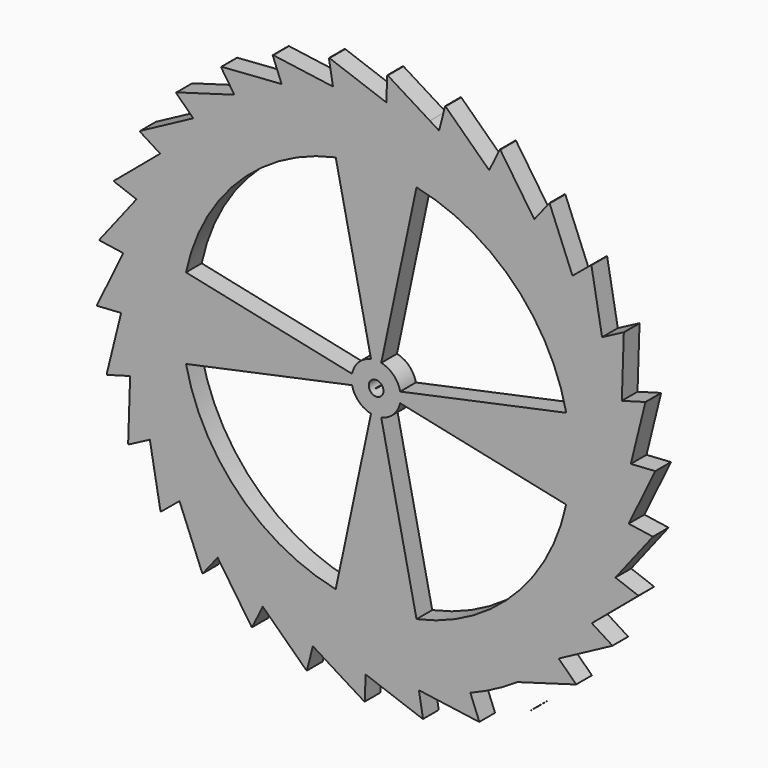
from build123d import *

# Parameters (mm, degrees)
F0_R     = 1.5
F1_DEPTH = 4


with BuildPart() as f1:
    # F0 (on Front) → F1 (new body)
    with BuildSketch(Plane.XZ):
        with BuildLine():
            ThreePointArc((51.423780965, -7.5173518176), (51.8332811532, -3.7685858239), (51.9700209308, 0))
            ThreePointArc((51.9700209308, 0), (51.9431469729, 1.6715769245), (51.8625528764, 3.3414260841))
            ThreePointArc((51.8625528764, 3.3414260841), (51.8624455569, 3.3430923455), (51.8623381838, 3.3447586034))
            ThreePointArc((51.8623381838, 3.3447586034), (51.2287251198, 8.7490139372), (50.0338550026, 14.0574719648))
            ThreePointArc((50.0338550026, 14.0574719648), (50.033403593, 14.0590795014), (50.0329521318, 14.0606870235))
            ThreePointArc((50.0329521318, 14.0606870235), (48.2895771693, 19.2151108485), (46.0171273468, 24.1591388654))
            ThreePointArc((46.0171273468, 24.1591388654), (46.0163515759, 24.1606174201), (46.0155757576, 24.1620959499))
            ThreePointArc((46.0155757576, 24.1620959499), (43.2386327482, 28.8414152114), (39.9879201821, 33.2049354692))
            ThreePointArc((39.9879201821, 33.2049354692), (39.9868539549, 33.2062204221), (39.9857876865, 33.2075053408))
            ThreePointArc((39.9857876865, 33.2075053408), (36.2966423649, 37.2072113331), (32.209738793, 40.799517058))
            ThreePointArc((32.209738793, 40.799517058), (32.2084287087, 40.8005522505), (32.2071185911, 40.801587401))
            ThreePointArc((32.2071185911, 40.801587401), (32.2038705968, 40.8041534125), (32.2006223982, 40.8067191655))
            ThreePointArc((32.2006223982, 40.8067191655), (27.7635059588, 43.9490863386), (23.02252703, 46.6109639736))
            ThreePointArc((23.02252703, 46.6109639736), (23.0210303455, 46.6117041628), (23.0195336373, 46.612444304))
            ThreePointArc((23.0195336373, 46.612444304), (18.0225046976, 48.7658469613), (12.8278101322, 50.3852880993))
            ThreePointArc((12.8278101322, 50.3852880993), (12.8261922599, 50.3857009355), (12.8245743743, 50.3861137196))
            ThreePointArc((12.8245743743, 50.3861137196), (11.8158452876, 50.6327605934), (10.8023920255, 50.8592148629))
            ThreePointArc((10.8023920255, 50.8592148629), (6.4600446281, 51.5934064819), (2.0711461478, 51.9575333597))
            ThreePointArc((2.0711461478, 51.9575333597), (2.0694777965, 51.9576007998), (2.0678094429, 51.9576681863))
            ThreePointArc((2.0678094429, 51.9576681863), (-3.3730714146, 51.892424626), (-8.7773470908, 51.2589850923))
            ThreePointArc((-8.7773470908, 51.2589850923), (-8.7789930063, 51.2587041889), (-8.7806389128, 51.2584232327))
            ThreePointArc((-8.7806389128, 51.2584232327), (-14.0890585705, 50.0633826621), (-19.2435383724, 48.3201732085))
            ThreePointArc((-19.2435383724, 48.3201732085), (-19.2450899176, 48.3195562385), (-19.246641443, 48.3189392186))
            ThreePointArc((-19.246641443, 48.3189392186), (-24.1905964893, 46.0463306451), (-28.8700049156, 43.2695378896))
            ThreePointArc((-28.8700049156, 43.2695378896), (-28.8713942805, 43.2686118174), (-28.8727836157, 43.2676857006))
            ThreePointArc((-28.8727836157, 43.2676857006), (-33.2361994913, 40.0168330241), (-37.2360239395, 36.3278161346))
            ThreePointArc((-37.2360239395, 36.3278161346), (-37.2371904022, 36.3266214341), (-37.2383568266, 36.3254266962))
            ThreePointArc((-37.2383568266, 36.3254266962), (-40.8305313197, 32.2384077779), (-43.9759602681, 27.7983944943))
            ThreePointArc((-43.9759602681, 27.7983944943), (-43.9768528486, 27.7969833797), (-43.9777453839, 27.7955722364))
            ThreePointArc((-43.9777453839, 27.7955722364), (-46.641683232, 23.0510094147), (-48.7952463421, 18.0540496231))
            ThreePointArc((-48.7952463421, 18.0540496231), (-48.7958260304, 18.0524837668), (-48.7964056684, 18.0509178919))
            ThreePointArc((-48.7964056684, 18.0509178919), (-50.4156800046, 12.8561713291), (-51.4832562346, 7.5206561505))
            ThreePointArc((-51.4832562346, 7.5206561505), (-51.4834976955, 7.5190039879), (-51.4837391033, 7.5173518176))
            ThreePointArc((-51.4837391033, 7.5173518176), (-51.9875798689, 2.0994568656), (-51.9225110148, -3.341426084))
            ThreePointArc((-51.9225110148, -3.341426084), (-51.9224036952, -3.3430923454), (-51.9222963221, -3.3447586034))
            ThreePointArc((-51.9222963221, -3.3447586034), (-51.2886832581, -8.7490139372), (-50.0938131409, -14.0574719648))
            ThreePointArc((-50.0938131409, -14.0574719648), (-50.0933617313, -14.0590795013), (-50.0929102701, -14.0606870234))
            ThreePointArc((-50.0929102701, -14.0606870234), (-48.3495353076, -19.2151108485), (-46.0770854851, -24.1591388654))
            ThreePointArc((-46.0770854851, -24.1591388654), (-46.0763097143, -24.1606174201), (-46.0755338959, -24.1620959499))
            ThreePointArc((-46.0755338959, -24.1620959499), (-43.2985908866, -28.8414152114), (-40.0478783205, -33.2049354692))
            ThreePointArc((-40.0478783205, -33.2049354692), (-40.0468120933, -33.2062204221), (-40.0457458248, -33.2075053408))
            ThreePointArc((-40.0457458248, -33.2075053408), (-36.3566005033, -37.207211333), (-32.2696969313, -40.799517058))
            ThreePointArc((-32.2696969313, -40.799517058), (-32.268386847, -40.8005522505), (-32.2670767295, -40.801587401))
            ThreePointArc((-32.2670767295, -40.801587401), (-27.8269624488, -43.9468737795), (-23.0824851683, -46.6109639736))
            ThreePointArc((-23.0824851683, -46.6109639736), (-23.0809884839, -46.6117041628), (-23.0794917756, -46.612444304))
            ThreePointArc((-23.0794917756, -46.612444304), (-18.082462836, -48.7658469613), (-12.8877682706, -50.3852880993))
            ThreePointArc((-12.8877682706, -50.3852880993), (-12.8861503982, -50.3857009355), (-12.8845325127, -50.3861137196))
            ThreePointArc((-12.8845325127, -50.3861137196), (-7.5489830571, -51.4535186263), (-2.1311042862, -51.9575333597))
            ThreePointArc((-2.1311042862, -51.9575333597), (-2.1294359348, -51.9576007998), (-2.1277675813, -51.9576681863))
            ThreePointArc((-2.1277675813, -51.9576681863), (3.3131132763, -51.892424626), (8.7173889525, -51.2589850923))
            ThreePointArc((8.7173889525, -51.2589850923), (8.719034868, -51.2587041889), (8.7206807744, -51.2584232327))
            ThreePointArc((8.7206807744, -51.2584232327), (14.0291004322, -50.0633826621), (19.1835802341, -48.3201732085))
            ThreePointArc((19.1835802341, -48.3201732085), (19.1851317793, -48.3195562385), (19.1866833047, -48.3189392186))
            ThreePointArc((19.1866833047, -48.3189392186), (24.1306383509, -46.0463306451), (28.8100467773, -43.2695378896))
            ThreePointArc((28.8100467773, -43.2695378896), (28.8114361422, -43.2686118174), (28.8128254774, -43.2676857007))
            ThreePointArc((28.8128254774, -43.2676857007), (33.1762413529, -40.0168330241), (37.1760658011, -36.3278161346))
            ThreePointArc((37.1760658011, -36.3278161346), (37.1772322639, -36.3266214341), (37.1783986882, -36.3254266962))
            ThreePointArc((37.1783986882, -36.3254266962), (40.7705731814, -32.2384077779), (43.9160021298, -27.7983944943))
            ThreePointArc((43.9160021298, -27.7983944943), (43.9168947103, -27.7969833797), (43.9177872455, -27.7955722364))
            ThreePointArc((43.9177872455, -27.7955722364), (46.5817250937, -23.0510094147), (48.7352882038, -18.0540496231))
            ThreePointArc((48.7352882038, -18.0540496231), (48.7358678921, -18.0524837668), (48.7364475301, -18.0509178919))
            ThreePointArc((48.7364475301, -18.0509178919), (50.3557218663, -12.8561713291), (51.4232980963, -7.5206561505))
            ThreePointArc((51.4232980963, -7.5206561505), (51.4235395572, -7.5190039879), (51.423780965, -7.5173518176))
        make_face()
        with BuildLine():
            Line((-38.7123002544, -8.1905973513), (-4.8907380037, -1.001602369))
            ThreePointArc((-4.8907380037, -1.001602369), (-3.535533906, -3.4975778209), (-1.0395584541, -4.8527819186))
            Line((-1.0395584541, -4.8527819186), (-8.2285534364, -38.6743441693))
            ThreePointArc((-8.2285534364, -38.6743441693), (-27.9852754377, -27.9473193526), (-38.7123002544, -8.1905973513))
        make_face(mode=Mode.SUBTRACT)
        with BuildLine():
            ThreePointArc((1.0395584541, -4.8527819186), (3.5201705738, -3.5128746813), (4.881539124, -1.0439754197))
            Line((4.881539124, -1.0439754197), (38.7032620429, -8.2330045531))
            ThreePointArc((38.7032620429, -8.2330045531), (27.9699412844, -27.9626451083), (8.2285534364, -38.6743441693))
            Line((8.2285534364, -38.6743441693), (1.0395584541, -4.8527819186))
        make_face(mode=Mode.SUBTRACT)
        with Locations((0, 0.037956085)):
            Circle(F0_R, mode=Mode.SUBTRACT)
        with BuildLine():
            ThreePointArc((-38.7212920003, 8.2240924432), (-28.0006011933, 28.0078973695), (-8.2285534364, 38.7502563394))
            Line((-8.2285534364, 38.7502563394), (-1.0395584541, 4.9286940887))
            ThreePointArc((-1.0395584541, 4.9286940887), (-3.5508307664, 3.5581266589), (-4.8995690813, 1.0350633097))
            Line((-4.8995690813, 1.0350633097), (-38.7212920003, 8.2240924432))
        make_face(mode=Mode.SUBTRACT)
        with BuildLine():
            ThreePointArc((4.8983222404, 1.0411705334), (3.5486358835, 3.5603392792), (1.0395584541, 4.9286940887))
            Line((1.0395584541, 4.9286940887), (8.2285534364, 38.7502563394))
            ThreePointArc((8.2285534364, 38.7502563394), (27.9983986149, 28.0101021886), (38.7200022863, 8.2301905538))
            Line((38.7200022863, 8.2301905538), (4.8983222404, 1.0411705334))
        make_face(mode=Mode.SUBTRACT)
        with BuildLine():
            ThreePointArc((51.8625528764, 3.3414260841), (51.9431469729, 1.6715769245), (51.9700209308, 0))
            ThreePointArc((51.9700209308, 0), (51.8332811532, -3.7685858239), (51.423780965, -7.5173518176))
            Line((51.423780965, -7.5173518176), (51.4248273891, -7.5175046993))
            Line((51.4248273891, -7.5175046993), (56.8415524882, 3.6448733841))
            ThreePointArc((56.8415524882, 3.6448733841), (56.8408849757, 3.6552424829), (56.8402155713, 3.6656114598))
            Line((56.8402155713, 3.6656114598), (51.863393527, 3.3448266263))
            Line((51.863393527, 3.3448266263), (51.8625528764, 3.3414260841))
        make_face()
        with BuildLine():
            ThreePointArc((51.8623381838, 3.3447586034), (51.8624455569, 3.3430923455), (51.8625528764, 3.3414260841))
            Line((51.8625528764, 3.3414260841), (51.863393527, 3.3448266263))
            Line((51.863393527, 3.3448266263), (51.8623381838, 3.3447586034))
        make_face()
        with BuildLine():
            Line((51.4248273891, -7.5175046993), (51.423780965, -7.5173518176))
            ThreePointArc((51.423780965, -7.5173518176), (51.4235395572, -7.5190039879), (51.4232980963, -7.5206561505))
            Line((51.4232980963, -7.5206561505), (51.4248273891, -7.5175046993))
        make_face()
        with BuildLine():
            ThreePointArc((50.0338550026, 14.0574719648), (51.2287251198, 8.7490139372), (51.8623381838, 3.3447586034))
            Line((51.8623381838, 3.3447586034), (51.863393527, 3.3448266263))
            Line((51.863393527, 3.3448266263), (54.8394310956, 15.383290621))
            ThreePointArc((54.8394310956, 15.383290621), (54.8358719487, 15.3959636245), (54.8323098726, 15.4086358049))
            Line((54.8323098726, 15.4086358049), (50.0339702704, 14.0609729781))
            Line((50.0339702704, 14.0609729781), (50.0338550025, 14.0574719648))
        make_face()
        with BuildLine():
            Line((51.4248273891, -7.5175046993), (51.4232980963, -7.5206561505))
            ThreePointArc((51.4232980963, -7.5206561505), (50.3557218663, -12.8561713291), (48.7364475301, -18.0509178919))
            Line((48.7364475301, -18.0509178919), (48.7374393014, -18.0512849966))
            Line((48.7374393014, -18.0512849966), (56.3583664405, -8.2567424152))
            ThreePointArc((56.3583664405, -8.2567424152), (56.3596879193, -8.2477096133), (56.3610079501, -8.2386765998))
            Line((56.3610079501, -8.2386765998), (51.4248273891, -7.5175046993))
        make_face()
        with BuildLine():
            ThreePointArc((50.0329521318, 14.0606870235), (50.033403593, 14.0590795014), (50.0338550026, 14.0574719648))
            Line((50.0338550025, 14.0574719648), (50.0339702704, 14.0609729781))
            Line((50.0339702704, 14.0609729781), (50.0329521318, 14.0606870235))
        make_face()
        with BuildLine():
            Line((48.7374393014, -18.0512849966), (48.7364475301, -18.0509178919))
            ThreePointArc((48.7364475301, -18.0509178919), (48.7358678921, -18.0524837668), (48.7352882038, -18.0540496231))
            Line((48.7352882038, -18.0540496231), (48.7374393014, -18.0512849966))
        make_face()
        with BuildLine():
            ThreePointArc((46.0171273468, 24.1591388654), (48.2895771693, 19.2151108485), (50.0329521318, 14.0606870235))
            Line((50.0329521318, 14.0606870235), (50.0339702704, 14.0609729781))
            Line((50.0339702704, 14.0609729781), (50.4417219085, 26.4455542565))
            ThreePointArc((50.4417219085, 26.4455542565), (50.4336714583, 26.4608959315), (50.425616341, 26.4762351567))
            Line((50.425616341, 26.4762351567), (46.0165121942, 24.1625873387))
            Line((46.0165121942, 24.1625873387), (46.0171273468, 24.1591388654))
        make_face()
        with BuildLine():
            Line((48.7374393014, -18.0512849966), (48.7352882038, -18.0540496231))
            ThreePointArc((48.7352882038, -18.0540496231), (46.5817250937, -23.0510094147), (43.9177872455, -27.7955722364))
            Line((43.9177872455, -27.7955722364), (43.918681019, -27.7961375198))
            Line((43.918681019, -27.7961375198), (53.4089351369, -19.8005617916))
            ThreePointArc((53.4089351369, -19.8005617916), (53.4122132861, -19.7917150962), (53.4154899695, -19.7828678578))
            Line((53.4154899695, -19.7828678579), (48.7374393014, -18.0512849966))
        make_face()
        with BuildLine():
            ThreePointArc((46.0155757576, 24.1620959499), (46.0163515759, 24.1606174201), (46.0171273468, 24.1591388654))
            Line((46.0171273468, 24.1591388654), (46.0165121942, 24.1625873387))
            Line((46.0165121942, 24.1625873387), (46.0155757576, 24.1620959499))
        make_face()
        with BuildLine():
            Line((43.918681019, -27.7961375198), (43.9177872455, -27.7955722364))
            ThreePointArc((43.9177872455, -27.7955722364), (43.9168947103, -27.7969833797), (43.9160021298, -27.7983944943))
            Line((43.9160021298, -27.7983944943), (43.918681019, -27.7961375198))
        make_face()
        with BuildLine():
            ThreePointArc((39.9879201821, 33.2049354692), (43.2386327482, 28.8414152114), (46.0155757576, 24.1620959499))
            Line((46.0155757576, 24.1620959499), (46.0165121942, 24.1625873387))
            Line((46.0165121942, 24.1625873387), (43.8426229041, 36.349154898))
            ThreePointArc((43.8426229041, 36.349154898), (43.8281298887, 36.3666205946), (43.8136299139, 36.384080514))
            Line((43.8136299139, 36.384080514), (39.9866014941, 33.2081806877))
            Line((39.9866014941, 33.2081806877), (39.9879201821, 33.2049354692))
        make_face()
        with BuildLine():
            Line((43.918681019, -27.7961375198), (43.9160021298, -27.7983944943))
            ThreePointArc((43.9160021298, -27.7983944943), (40.7705731814, -32.2384077779), (37.1783986882, -36.3254266962))
            Line((37.1783986883, -36.3254266962), (37.1791554016, -36.3261654528))
            Line((37.1791554016, -36.3261654528), (48.1206244533, -30.4804633073))
            ThreePointArc((48.1206244533, -30.4804633073), (48.1266672862, -30.4709204774), (48.1327082262, -30.4613764493))
            Line((48.1327082262, -30.4613764493), (43.918681019, -27.7961375198))
        make_face()
        with BuildLine():
            ThreePointArc((39.9857876865, 33.2075053408), (39.9868539549, 33.2062204221), (39.9879201821, 33.2049354692))
            Line((39.9879201821, 33.2049354692), (39.9866014941, 33.2081806877))
            Line((39.9866014941, 33.2081806877), (39.9857876865, 33.2075053408))
        make_face()
        with BuildLine():
            Line((37.1791554016, -36.3261654528), (37.1783986883, -36.3254266962))
            ThreePointArc((37.1783986882, -36.3254266962), (37.1772322639, -36.3266214341), (37.1760658011, -36.3278161346))
            Line((37.1760658011, -36.3278161346), (37.1791554016, -36.3261654528))
        make_face()
        with BuildLine():
            ThreePointArc((32.209738793, 40.799517058), (36.2966423649, 37.2072113331), (39.9857876865, 33.2075053408))
            Line((39.9857876865, 33.2075053408), (39.9866014941, 33.2081806877))
            Line((39.9866014941, 33.2081806877), (35.3319790375, 44.662949992))
            ThreePointArc((35.3319790375, 44.662949992), (35.3091952691, 44.6809558924), (35.286402322, 44.6989501724))
            Line((35.286402322, 44.6989501724), (32.2091226063, 40.8041238266))
            Line((32.2091226063, 40.8041238266), (32.209738793, 40.799517058))
        make_face()
        with BuildLine():
            Line((37.1791554016, -36.3261654528), (37.1760658011, -36.3278161346))
            ThreePointArc((37.1760658011, -36.3278161346), (33.1762413529, -40.0168330241), (28.8128254774, -43.2676857007))
            Line((28.8128254774, -43.2676857007), (28.8134120585, -43.2685656432))
            Line((28.8134120585, -43.2685656432), (40.7238038627, -39.8275945924))
            ThreePointArc((40.7238038627, -39.8275945924), (40.7340326593, -39.8171332475), (40.7442587679, -39.8066692749))
            Line((40.7442587679, -39.8066692749), (37.1791554016, -36.3261654528))
        make_face()
        with BuildLine():
            ThreePointArc((32.2071185911, 40.801587401), (32.2084287087, 40.8005522505), (32.209738793, 40.799517058))
            Line((32.209738793, 40.799517058), (32.2077742026, 40.80241719))
            Line((32.2077742026, 40.80241719), (32.2071185911, 40.801587401))
        make_face()
        Polygon((32.2077742026, 40.80241719), (32.209738793, 40.799517058), (32.2091226063, 40.8041238266), align=None)
        with BuildLine():
            Line((28.8134120585, -43.2685656432), (28.8128254774, -43.2676857007))
            ThreePointArc((28.8128254774, -43.2676857007), (28.8114361422, -43.2686118174), (28.8100467773, -43.2695378896))
            Line((28.8100467773, -43.2695378896), (28.8134120585, -43.2685656432))
        make_face()
        with BuildLine():
            ThreePointArc((32.2006223982, 40.8067191655), (32.2038705968, 40.8041534125), (32.2071185911, 40.801587401))
            Line((32.2071185911, 40.801587401), (32.2077742026, 40.80241719))
            Line((32.2077742026, 40.80241719), (32.2029035341, 40.8096072802))
            Line((32.2029035341, 40.8096072802), (32.2006223982, 40.8067191655))
        make_face()
        Polygon((32.2029035341, 40.8096072802), (32.2077742026, 40.80241719), (32.2091226063, 40.8041238266), (32.2075947163, 40.8155467211), align=None)
        with BuildLine():
            ThreePointArc((23.02252703, 46.6109639736), (27.7635059588, 43.9490863386), (32.2006223982, 40.8067191655))
            Line((32.2006223982, 40.8067191655), (32.2029035341, 40.8096072802))
            Line((32.2029035341, 40.8096072802), (25.282367975, 51.0257149897))
            ThreePointArc((25.282367975, 51.0257149897), (25.2500286651, 51.0417168963), (25.2176792232, 51.0576983102))
            Line((25.2176792232, 51.0576983102), (23.0200023993, 46.6133922695))
            Line((23.0200023993, 46.6133922695), (23.02252703, 46.6109639736))
        make_face()
        with BuildLine():
            Line((19.1870741173, -48.3199218894), (19.1866833047, -48.3189392186))
            ThreePointArc((19.1866833047, -48.3189392186), (19.1851317793, -48.3195562385), (19.1835802341, -48.3201732085))
            Line((19.1835802341, -48.3201732085), (19.1870741173, -48.3199218894))
        make_face()
        with BuildLine():
            ThreePointArc((23.0195336373, 46.612444304), (23.0210303455, 46.6117041628), (23.02252703, 46.6109639736))
            Line((23.02252703, 46.6109639736), (23.0200023993, 46.6133922695))
            Line((23.0200023993, 46.6133922695), (23.0195336373, 46.612444304))
        make_face()
        with BuildLine():
            Line((19.1870741173, -48.3199218894), (19.1835802341, -48.3201732085))
            ThreePointArc((19.1835802341, -48.3201732085), (14.0291004322, -50.0633826621), (8.7206807744, -51.2584232327))
            Line((8.7206807744, -51.2584232327), (8.7208587382, -51.2594656842))
            Line((8.7208587382, -51.2594656842), (20.9772836713, -52.9570745732))
            ThreePointArc((20.9772836713, -52.9570745732), (21.0006110859, -52.9478310737), (21.0239344255, -52.9385772969))
            Line((21.0239344255, -52.9385772969), (19.1870741173, -48.3199218894))
        make_face()
        with BuildLine():
            ThreePointArc((12.8278101322, 50.3852880993), (18.0225046976, 48.7658469613), (23.0195336373, 46.612444304))
            Line((23.0195336373, 46.612444304), (23.0200023993, 46.6133922695))
            Line((23.0200023993, 46.6133922695), (14.1327095736, 55.1615638726))
            ThreePointArc((14.1327095736, 55.1615638726), (14.0905496682, 55.1723391221), (14.0483815417, 55.1830821538))
            Line((14.0483815417, 55.1830821538), (12.8248357996, 50.3871384309))
            Line((12.8248357996, 50.3871384309), (12.8278101322, 50.3852880993))
        make_face()
        with BuildLine():
            Line((8.7208587382, -51.2594656842), (8.7206807744, -51.2584232327))
            ThreePointArc((8.7206807744, -51.2584232327), (8.719034868, -51.2587041889), (8.7173889525, -51.2589850923))
            Line((8.7173889525, -51.2589850923), (8.7208587382, -51.2594656842))
        make_face()
        with BuildLine():
            ThreePointArc((12.8245743743, 50.3861137196), (12.8261922599, 50.3857009355), (12.8278101322, 50.3852880993))
            Line((12.8278101322, 50.3852880993), (12.8248357996, 50.3871384309))
            Line((12.8248357996, 50.3871384309), (12.8245743743, 50.3861137196))
        make_face()
        with BuildLine():
            Line((8.7208587382, -51.2594656842), (8.7173889525, -51.2589850923))
            ThreePointArc((8.7173889525, -51.2589850923), (3.3131132763, -51.892424626), (-2.1277675813, -51.9576681863))
            Line((-2.1277675813, -51.9576681863), (-2.1278102444, -51.9587248585))
            Line((-2.1278102444, -51.9587248585), (9.4934072875, -56.1622741859))
            ThreePointArc((9.4934072875, -56.1622741859), (9.5247237806, -56.1569763154), (9.5560373141, -56.1516609799))
            Line((9.5560373141, -56.1516609799), (8.7208587382, -51.2594656842))
        make_face()
        with BuildLine():
            ThreePointArc((10.8023920255, 50.8592148629), (11.8158452876, 50.6327605934), (12.8245743743, 50.3861137196))
            Line((12.8245743743, 50.3861137196), (12.8248357996, 50.3871384309))
            Line((12.8248357996, 50.3871384309), (10.949965744, 51.5534946223))
            Line((10.949965744, 51.5534946223), (10.8023920255, 50.8592148629))
        make_face()
        with BuildLine():
            Line((-2.1278102444, -51.9587248585), (-2.1277675813, -51.9576681863))
            ThreePointArc((-2.1277675813, -51.9576681863), (-2.1294359348, -51.9576007998), (-2.1311042862, -51.9575333597))
            Line((-2.1311042862, -51.9575333597), (-2.1278102444, -51.9587248585))
        make_face()
        with BuildLine():
            ThreePointArc((2.0711461478, 51.9575333597), (6.4600446281, 51.5934064819), (10.8023920255, 50.8592148629))
            Line((10.8023920255, 50.8592148629), (10.949965744, 51.5534946223))
            Line((10.949965744, 51.5534946223), (2.3691338098, 56.8916280168))
            ThreePointArc((2.3691338098, 56.8916280168), (2.318160244, 56.8937186784), (2.2671848258, 56.8957636756))
            Line((2.2671848258, 56.8957636756), (2.067852106, 51.9587248585))
            Line((2.067852106, 51.9587248585), (2.0711461478, 51.9575333597))
        make_face()
        with BuildLine():
            Line((-2.1278102444, -51.9587248585), (-2.1311042862, -51.9575333597))
            ThreePointArc((-2.1311042862, -51.9575333597), (-7.5489830571, -51.4535186263), (-12.8845325127, -50.3861137196))
            Line((-12.8845325127, -50.3861137196), (-12.884793938, -50.3871384309))
            Line((-12.884793938, -50.3871384309), (-2.4056567842, -56.9062070265))
            ThreePointArc((-2.4056567842, -56.9062070265), (-2.3666769917, -56.9078484907), (-2.3276960839, -56.9094632505))
            Line((-2.3276960839, -56.9094632505), (-2.1278102444, -51.9587248585))
        make_face()
        with BuildLine():
            ThreePointArc((2.0678094429, 51.9576681863), (2.0694777965, 51.9576007998), (2.0711461478, 51.9575333597))
            Line((2.0711461478, 51.9575333597), (2.067852106, 51.9587248585))
            Line((2.067852106, 51.9587248585), (2.0678094429, 51.9576681863))
        make_face()
        with BuildLine():
            Line((-12.884793938, -50.3871384309), (-12.8845325127, -50.3861137196))
            ThreePointArc((-12.8845325127, -50.3861137196), (-12.8861503982, -50.3857009355), (-12.8877682706, -50.3852880993))
            Line((-12.8877682706, -50.3852880993), (-12.884793938, -50.3871384309))
        make_face()
        with BuildLine():
            ThreePointArc((-8.7773470908, 51.2589850923), (-3.3730714146, 51.892424626), (2.0678094429, 51.9576681863))
            Line((2.0678094429, 51.9576681863), (2.067852106, 51.9587248585))
            Line((2.067852106, 51.9587248585), (-9.4960653121, 56.1415479707))
            ThreePointArc((-9.4960653121, 56.1415479707), (-9.553501977, 56.1317939904), (-9.6109286334, 56.1219812573))
            Line((-9.6109286334, 56.1219812573), (-8.7808168765, 51.2594656842))
            Line((-8.7808168765, 51.2594656842), (-8.7773470908, 51.2589850923))
        make_face()
        with BuildLine():
            Line((-12.884793938, -50.3871384309), (-12.8877682706, -50.3852880993))
            ThreePointArc((-12.8877682706, -50.3852880993), (-18.082462836, -48.7658469613), (-23.0794917756, -46.612444304))
            Line((-23.0794917756, -46.612444304), (-23.0799605376, -46.6133922695))
            Line((-23.0799605376, -46.6133922695), (-14.1976694582, -55.1567529829))
            ThreePointArc((-14.1976694582, -55.1567529829), (-14.1526030357, -55.1683435564), (-14.1075271576, -55.1798973022))
            Line((-14.1075271576, -55.1798973022), (-12.884793938, -50.3871384309))
        make_face()
        with BuildLine():
            ThreePointArc((-8.7806389128, 51.2584232327), (-8.7789930063, 51.2587041889), (-8.7773470908, 51.2589850923))
            Line((-8.7773470908, 51.2589850923), (-8.7808168765, 51.2594656842))
            Line((-8.7808168765, 51.2594656842), (-8.7806389128, 51.2584232327))
        make_face()
        with BuildLine():
            Line((-23.0799605376, -46.6133922695), (-23.0794917756, -46.612444304))
            ThreePointArc((-23.0794917756, -46.612444304), (-23.0809884839, -46.6117041628), (-23.0824851683, -46.6109639736))
            Line((-23.0824851683, -46.6109639736), (-23.0799605376, -46.6133922695))
        make_face()
        with BuildLine():
            ThreePointArc((-19.2435383724, 48.3201732085), (-14.0890585705, 50.0633826621), (-8.7806389128, 51.2584232327))
            Line((-8.7806389128, 51.2584232327), (-8.7808168765, 51.2594656842))
            Line((-8.7808168765, 51.2594656842), (-20.9465042524, 52.9445067253))
            ThreePointArc((-20.9465042524, 52.9445067253), (-21.0068617668, 52.9205801703), (-21.0671919636, 52.8965848179))
            Line((-21.0671919636, 52.8965848179), (-19.2470322556, 48.3199218893))
            Line((-19.2470322556, 48.3199218893), (-19.2435383724, 48.3201732085))
        make_face()
        with BuildLine():
            Line((-23.0799605376, -46.6133922695), (-23.0824851683, -46.6109639736))
            ThreePointArc((-23.0824851683, -46.6109639736), (-27.8269624488, -43.9468737795), (-32.2670767295, -40.801587401))
            Line((-32.2670767295, -40.801587401), (-32.267732341, -40.80241719))
            Line((-32.267732341, -40.80241719), (-25.3654197169, -50.9916241683))
            ThreePointArc((-25.3654197169, -50.9916241683), (-25.3170761133, -51.0156571166), (-25.2687097482, -51.0396442242))
            Line((-25.2687097482, -51.0396442242), (-23.0799605376, -46.6133922695))
        make_face()
        with BuildLine():
            ThreePointArc((-19.246641443, 48.3189392186), (-19.2450899176, 48.3195562385), (-19.2435383724, 48.3201732085))
            Line((-19.2435383724, 48.3201732085), (-19.2470322556, 48.3199218893))
            Line((-19.2470322556, 48.3199218893), (-19.246641443, 48.3189392186))
        make_face()
        with BuildLine():
            Line((-32.267732341, -40.80241719), (-32.2670767295, -40.801587401))
            ThreePointArc((-32.2670767295, -40.801587401), (-32.268386847, -40.8005522505), (-32.2696969313, -40.799517058))
            Line((-32.2696969314, -40.799517058), (-32.267732341, -40.80241719))
        make_face()
        with BuildLine():
            ThreePointArc((-28.8700049156, 43.2695378896), (-24.1905964893, 46.0463306451), (-19.246641443, 48.3189392186))
            Line((-19.246641443, 48.3189392186), (-19.2470322556, 48.3199218893))
            Line((-19.2470322556, 48.3199218893), (-31.4839020622, 47.4397093574))
            ThreePointArc((-31.4839020622, 47.4397093574), (-31.5428070152, 47.4005584273), (-31.6016632984, 47.3613343691))
            Line((-31.6016632984, 47.3613343691), (-28.8733701969, 43.2685656432))
            Line((-28.8733701969, 43.2685656432), (-28.8700049156, 43.2695378896))
        make_face()
        with BuildLine():
            Line((-32.267732341, -40.80241719), (-32.2696969314, -40.799517058))
            ThreePointArc((-32.2696969313, -40.799517058), (-36.3566005033, -37.207211333), (-40.0457458248, -33.2075053408))
            Line((-40.0457458248, -33.2075053408), (-40.0465596325, -33.2081806877))
            Line((-40.0465596325, -33.2081806877), (-35.4196493073, -44.5947519638))
            ThreePointArc((-35.4196493073, -44.5947519638), (-35.3718307251, -44.6327081594), (-35.3239714799, -44.6706130698))
            Line((-35.3239714799, -44.6706130698), (-32.267732341, -40.80241719))
        make_face()
        with BuildLine():
            ThreePointArc((-28.8727836157, 43.2676857006), (-28.8713942805, 43.2686118174), (-28.8700049156, 43.2695378896))
            Line((-28.8700049156, 43.2695378896), (-28.8733701969, 43.2685656432))
            Line((-28.8733701969, 43.2685656432), (-28.8727836157, 43.2676857006))
        make_face()
        with BuildLine():
            Line((-40.0465596325, -33.2081806877), (-40.0457458248, -33.2075053408))
            ThreePointArc((-40.0457458248, -33.2075053408), (-40.0468120933, -33.2062204221), (-40.0478783205, -33.2049354692))
            Line((-40.0478783205, -33.2049354692), (-40.0465596325, -33.2081806877))
        make_face()
        with BuildLine():
            ThreePointArc((-37.2360239395, 36.3278161346), (-33.2361994913, 40.0168330241), (-28.8727836157, 43.2676857006))
            Line((-28.8727836157, 43.2676857006), (-28.8733701969, 43.2685656432))
            Line((-28.8733701969, 43.2685656432), (-40.6494848981, 39.866387911))
            ThreePointArc((-40.6494848981, 39.866387911), (-40.702250937, 39.8125124482), (-40.7549455886, 39.7585671606))
            Line((-40.7549455886, 39.7585671606), (-37.2391135399, 36.3261654528))
            Line((-37.2391135399, 36.3261654528), (-37.2360239395, 36.3278161346))
        make_face()
        with BuildLine():
            Line((-40.0465596325, -33.2081806877), (-40.0478783205, -33.2049354692))
            ThreePointArc((-40.0478783205, -33.2049354692), (-43.2985908866, -28.8414152114), (-46.0755338959, -24.1620959499))
            Line((-46.0755338959, -24.1620959499), (-46.0764703325, -24.1625873387))
            Line((-46.0764703325, -24.1625873387), (-43.9206397604, -36.2479198503))
            ThreePointArc((-43.9206397604, -36.2479198503), (-43.8777101404, -36.2998976723), (-43.8347190213, -36.3518246394))
            Line((-43.8347190213, -36.3518246394), (-40.0465596325, -33.2081806877))
        make_face()
        with BuildLine():
            ThreePointArc((-37.2383568266, 36.3254266962), (-37.2371904022, 36.3266214341), (-37.2360239395, 36.3278161346))
            Line((-37.2360239395, 36.3278161346), (-37.2391135399, 36.3261654528))
            Line((-37.2391135399, 36.3261654528), (-37.2383568266, 36.3254266962))
        make_face()
        with BuildLine():
            Line((-46.0764703325, -24.1625873387), (-46.0755338959, -24.1620959499))
            ThreePointArc((-46.0755338959, -24.1620959499), (-46.0763097143, -24.1606174201), (-46.0770854851, -24.1591388654))
            Line((-46.0770854851, -24.1591388654), (-46.0764703325, -24.1625873387))
        make_face()
        with BuildLine():
            ThreePointArc((-43.9759602681, 27.7983944943), (-40.8305313197, 32.2384077779), (-37.2383568266, 36.3254266962))
            Line((-37.2383568266, 36.3254266962), (-37.2391135399, 36.3261654528))
            Line((-37.2391135399, 36.3261654528), (-48.0437317347, 30.553578658))
            ThreePointArc((-48.0437317347, 30.553578658), (-48.0859568135, 30.4870854322), (-48.1280898835, 30.4205338674))
            Line((-48.1280898835, 30.4205338674), (-43.9786391573, 27.7961375198))
            Line((-43.9786391573, 27.7961375198), (-43.9759602681, 27.7983944943))
        make_face()
        with BuildLine():
            Line((-46.0764703325, -24.1625873387), (-46.0770854851, -24.1591388654))
            ThreePointArc((-46.0770854851, -24.1591388654), (-48.3495353076, -19.2151108485), (-50.0929102701, -14.0606870234))
            Line((-50.0929102701, -14.0606870234), (-50.0939284087, -14.0609729781))
            Line((-50.0939284087, -14.0609729781), (-50.4974825669, -26.3180648082))
            ThreePointArc((-50.4974825669, -26.3180648082), (-50.4638106521, -26.3826051244), (-50.4300562652, -26.4471023462))
            Line((-50.4300562652, -26.4471023462), (-46.0764703325, -24.1625873387))
        make_face()
        with BuildLine():
            ThreePointArc((-43.9777453839, 27.7955722364), (-43.9768528486, 27.7969833797), (-43.9759602681, 27.7983944943))
            Line((-43.9759602681, 27.7983944943), (-43.9786391573, 27.7961375198))
            Line((-43.9786391573, 27.7961375198), (-43.9777453839, 27.7955722364))
        make_face()
        with BuildLine():
            Line((-50.0939284087, -14.0609729781), (-50.0929102701, -14.0606870234))
            ThreePointArc((-50.0929102701, -14.0606870234), (-50.0933617313, -14.0590795013), (-50.0938131409, -14.0574719648))
            Line((-50.0938131409, -14.0574719648), (-50.0939284087, -14.0609729781))
        make_face()
        with BuildLine():
            ThreePointArc((-48.7952463421, 18.0540496231), (-46.641683232, 23.0510094147), (-43.9777453839, 27.7955722364))
            Line((-43.9777453839, 27.7955722364), (-43.9786391573, 27.7961375198))
            Line((-43.9786391573, 27.7961375198), (-53.3436511702, 19.9060787485))
            ThreePointArc((-53.3436511702, 19.9060787485), (-53.3718003067, 19.8305004484), (-53.3998423824, 19.7548823596))
            Line((-53.3998423824, 19.7548823596), (-48.7973974398, 18.0512849966))
            Line((-48.7973974398, 18.0512849966), (-48.7952463421, 18.0540496231))
        make_face()
        with BuildLine():
            Line((-50.0939284087, -14.0609729781), (-50.0938131409, -14.0574719648))
            ThreePointArc((-50.0938131409, -14.0574719648), (-51.2886832581, -8.7490139372), (-51.9222963221, -3.3447586034))
            Line((-51.9222963221, -3.3447586034), (-51.9233516653, -3.3448266263))
            Line((-51.9233516653, -3.3448266263), (-54.8641810897, -15.2408690398))
            ThreePointArc((-54.8641810897, -15.2408690398), (-54.8435457723, -15.3150124413), (-54.8228102756, -15.3891278884))
            Line((-54.8228102756, -15.3891278884), (-50.0939284087, -14.0609729781))
        make_face()
        with BuildLine():
            ThreePointArc((-48.7964056684, 18.0509178919), (-48.7958260304, 18.0524837668), (-48.7952463421, 18.0540496231))
            Line((-48.7952463421, 18.0540496231), (-48.7973974398, 18.0512849966))
            Line((-48.7973974398, 18.0512849966), (-48.7964056684, 18.0509178919))
        make_face()
        with BuildLine():
            Line((-51.9233516653, -3.3448266263), (-51.9222963221, -3.3447586034))
            ThreePointArc((-51.9222963221, -3.3447586034), (-51.9224036952, -3.3430923454), (-51.9225110148, -3.341426084))
            Line((-51.9225110148, -3.341426084), (-51.9233516653, -3.3448266263))
        make_face()
        with BuildLine():
            ThreePointArc((-51.4832562346, 7.5206561505), (-50.4156800046, 12.8561713291), (-48.7964056684, 18.0509178919))
            Line((-48.7964056684, 18.0509178919), (-48.7973974398, 18.0512849966))
            Line((-48.7973974398, 18.0512849966), (-56.3168665037, 8.3871380244))
            ThreePointArc((-56.3168665037, 8.3871380244), (-56.3287472512, 8.3070387333), (-56.3405140937, 8.2269226299))
            Line((-56.3405140937, 8.2269226299), (-51.4847855274, 7.5175046993))
            Line((-51.4847855274, 7.5175046993), (-51.4832562346, 7.5206561505))
        make_face()
        with BuildLine():
            Line((-51.9233516653, -3.3448266263), (-51.9225110148, -3.341426084))
            ThreePointArc((-51.9225110148, -3.341426084), (-51.9875798689, 2.0994568656), (-51.4837391033, 7.5173518176))
            Line((-51.4837391033, 7.5173518176), (-51.4847855274, 7.5175046993))
            Line((-51.4847855274, 7.5175046993), (-56.8318994083, -3.5014238418))
            ThreePointArc((-56.8318994083, -3.5014238418), (-56.8269535962, -3.5809984397), (-56.8218963851, -3.6605660356))
            Line((-56.8218963851, -3.6605660356), (-51.9233516653, -3.3448266263))
        make_face()
        with BuildLine():
            ThreePointArc((-51.4837391033, 7.5173518176), (-51.4834976955, 7.5190039879), (-51.4832562346, 7.5206561505))
            Line((-51.4832562346, 7.5206561505), (-51.4847855274, 7.5175046993))
            Line((-51.4847855274, 7.5175046993), (-51.4837391033, 7.5173518176))
        make_face()
    extrude(amount=F1_DEPTH)


with BuildPart() as f1b:
    # F0 (on Front) → F1, piece 2 (new body)
    with BuildSketch(Plane.XZ):
        with BuildLine():
            Line((35.286402322, 44.6989501724), (35.30683952, 44.7248169588))
            ThreePointArc((35.30683952, 44.7248169588), (35.304875226, 44.7296501316), (35.3029103418, 44.7344830645))
            Line((35.3029103418, 44.7344830645), (35.2792820088, 44.7045675587))
            ThreePointArc((35.2792820088, 44.7045675587), (35.2828422773, 44.7017590073), (35.286402322, 44.6989501724))
        make_face()
    extrude(amount=F1_DEPTH)


with BuildPart() as f1c:
    # F0 (on Front) → F1, piece 3 (new body)
    with BuildSketch(Plane.XZ):
        with BuildLine():
            Line((31.5861720684, -47.428040095), (31.5740417975, -47.4098432256))
            ThreePointArc((31.5740417975, -47.4098432256), (31.5579776151, -47.4205363006), (31.5419098102, -47.4312239316))
            Line((31.5419098102, -47.4312239316), (31.5861720684, -47.428040095))
        make_face()
    extrude(amount=F1_DEPTH)


with BuildPart() as f1d:
    # F0 (on Front) → F1, piece 4 (new body)
    with BuildSketch(Plane.XZ):
        Polygon((0.0077190653, 0.001640738), (0, 0), (-0.008067815, 0), (-0.0090149787, -0.004456055), (0.0098681227, -0.0084697821), align=None)
        Polygon((-0.008067815, 0), (0, 0), (0.0077190653, 0.001640738), (0, 0.037956085), align=None)
        Polygon((-0.0090149787, -0.004456055), (-0.008067815, 0), (-0.0299790692, 0), align=None)
        Polygon((-0.0299790692, 0), (-0.008067815, 0), (0, 0.037956085), align=None)
        Polygon((-0.1042742049, 0.0157919186), (-0.0299790692, 0), (0, 0.037956085), align=None)
    extrude(amount=F1_DEPTH)


solid = Compound([f1.part, f1b.part, f1c.part, f1d.part])
